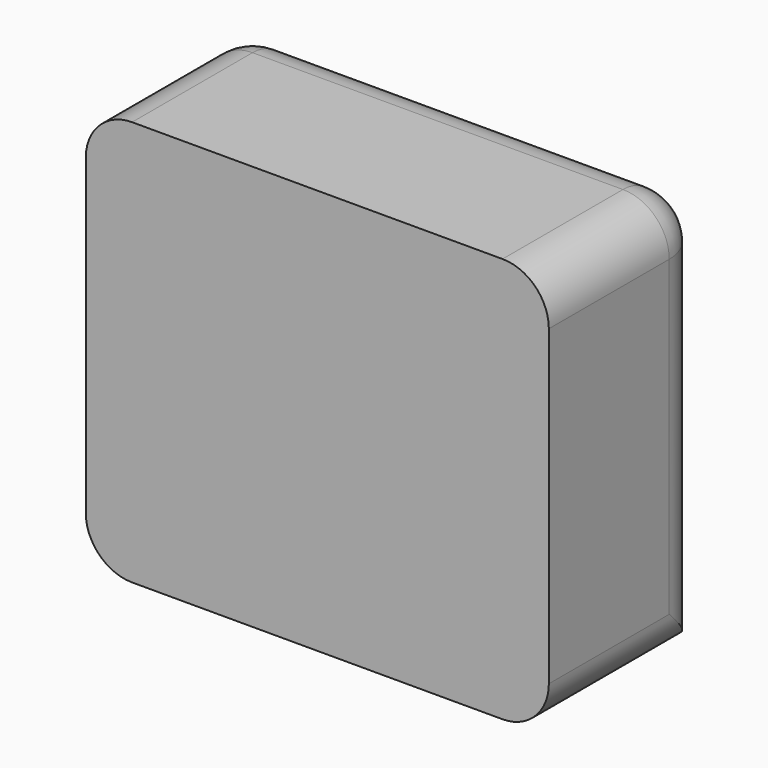
from build123d import *

# Parameters (mm, degrees)
F0_W         = 50.8
F0_H         = 44.45
F0_W_2       = 19.05
F0_H_2       = 5.08
F0_W_3       = 21.6944364339
F0_H_3       = 5.4140361476
F1_DEPTH     = 10.795
F2_W         = 50.8
F2_H         = 44.45
F3_DEPTH     = 3.81
F4_R         = 5.08
F5_SIZE      = 1.27
F6_R         = 2.54
F7_R         = 2.53999
F8_T1_DEPTH  = 52.07
F8_T3_DEPTH  = 46.99
F8_T5_DEPTH  = 40.64
F8_T8_ANGLE  = 90
F8_T10_ANGLE = 90


# Not quite as in the source:
# - a fillet or chamfer that OpenCascade refuses, or shapes differently, is made with other operations: its cross-section is extruded or revolved along the edge and cut away or added
# - a fillet or chamfer is up to 0.001 mm smaller than in the source, because OpenCascade refuses the exact size


with BuildPart() as f1:
    # F0 (on Front) → F1 (new body, symmetric)
    with BuildSketch(Plane.XZ):
        Rectangle(F0_W, F0_H)
        with Locations((-11.4416993469, -16.6936574811)):
            Rectangle(F0_W_2, F0_H_2, mode=Mode.SUBTRACT)
        with Locations((-11.4416993469, -9.0736574811)):
            Rectangle(F0_W_2, F0_H_2, mode=Mode.SUBTRACT)
        with Locations((-11.4416993469, -1.4536574811)):
            Rectangle(F0_W_2, F0_H_2, mode=Mode.SUBTRACT)
        with Locations((11.4416993469, -16.6936574811)):
            Rectangle(F0_W_2, F0_H_2, mode=Mode.SUBTRACT)
        with Locations((11.4416993469, -9.0736574811)):
            Rectangle(F0_W_2, F0_H_2, mode=Mode.SUBTRACT)
        with Locations((11.4416993469, -1.4536574811)):
            Rectangle(F0_W_2, F0_H_2, mode=Mode.SUBTRACT)
        with Locations((-11.4416993469, 6.1663425189)):
            Rectangle(F0_W_2, F0_H_2, mode=Mode.SUBTRACT)
        with Locations((-12.7639175639, 14.6224689895)):
            Rectangle(F0_W_3, F0_H_3, mode=Mode.SUBTRACT)
        with Locations((11.4416993469, 6.1663425189)):
            Rectangle(F0_W_2, F0_H_2, mode=Mode.SUBTRACT)
        with Locations((12.7639175639, 14.6224689895)):
            Rectangle(F0_W_3, F0_H_3, mode=Mode.SUBTRACT)
    extrude(amount=F1_DEPTH, both=True)

    # F2 (on face) → F3 (join)
    with BuildSketch(Plane.XZ.offset(10.795)):
        Rectangle(F2_W, F2_H)
    extrude(amount=-F3_DEPTH)

    # F4
    f4_edges = [f1.edges().sort_by_distance(p)[0] for p in [
        (25.4, 0, 22.225),
        (-25.4, 0, 22.225),
    ]]
    fillet(f4_edges, radius=F4_R)

    # F5
    f5_edges = [f1.edges().sort_by_distance(p)[0] for p in [
        (12.763918, 10.795, 11.915451),
        (-12.763918, 10.795, 11.915451),
        (-11.441699, 10.795, 3.626343),
        (11.441699, 10.795, 3.626343),
        (11.441699, 10.795, -3.993657),
        (-11.441699, 10.795, -3.993657),
        (-11.441699, 10.795, -11.613657),
        (11.441699, 10.795, -11.613657),
        (11.441699, 10.795, -19.233657),
        (-11.441699, 10.795, -19.233657),
    ]]
    chamfer(f5_edges, length=F5_SIZE)

    # F6
    f6_edges = [f1.edges().sort_by_distance(p)[0] for p in [
        (11.441699, -6.985, 3.626343),
        (-11.441699, -6.985, 3.626343),
        (-12.763918, -6.985, 11.915451),
        (12.763918, -6.985, 11.915451),
        (11.441699, -6.985, -3.993657),
        (-11.441699, -6.985, -3.993657),
        (11.441699, -6.985, -11.613657),
        (-11.441699, -6.985, -11.613657),
        (11.441699, -6.985, -19.233657),
        (-11.441699, -6.985, -19.233657),
    ]]
    fillet(f6_edges, radius=F6_R)

    # F7 (radius 2.54 in the source; OpenCascade refuses exactly that, so slightly less here)
    f7_edges = [f1.edges().sort_by_distance(p)[0] for p in [
        (11.441699, -6.985, 1.086343),
        (11.441699, -6.985, 8.706343),
        (-11.441699, -6.985, 8.706343),
        (-11.441699, -6.985, 1.086343),
        (-11.441699, -6.985, -6.533657),
        (11.441699, -6.985, -6.533657),
        (-12.763918, -6.985, 17.329487),
        (12.763918, -6.985, 17.329487),
        (11.441699, -6.985, -14.153657),
        (-11.441699, -6.985, -14.153657),
    ]]
    fillet(f7_edges, radius=F7_R)

    # F8: fillet of radius 5.08 on 4 edges, made by hand

    # F8_s2 → F8_t1 (cut)
    with BuildSketch(Plane.XY.offset(-34.925)):
        with BuildLine():
            ThreePointArc((20.32, 10.795), (23.9121024484, 9.3071024484), (25.4, 5.715))
            Line((25.4, 5.715), (25.4, 10.795))
            Line((25.4, 10.795), (20.32, 10.795))
        make_face()
        with BuildLine():
            ThreePointArc((-20.32, 10.795), (-23.9121024484, 9.3071024484), (-25.4, 5.715))
            Line((-25.4, 5.715), (-25.4, 10.795))
            Line((-25.4, 10.795), (-20.32, 10.795))
        make_face()
    extrude(amount=F8_T1_DEPTH, mode=Mode.SUBTRACT)

    # F8_s4 → F8_t3 (cut)
    with BuildSketch(Plane.XZ.offset(-23.495)):
        with BuildLine():
            ThreePointArc((-25.4, -17.145), (-23.9121024484, -20.7371024484), (-20.32, -22.225))
            Line((-20.32, -22.225), (-25.4, -22.225))
            Line((-25.4, -22.225), (-25.4, -17.145))
        make_face()
        with BuildLine():
            ThreePointArc((20.32, -22.225), (23.9121024484, -20.7371024484), (25.4, -17.145))
            Line((25.4, -17.145), (25.4, -22.225))
            Line((25.4, -22.225), (20.32, -22.225))
        make_face()
    extrude(amount=F8_T3_DEPTH, mode=Mode.SUBTRACT)

    # F8_s6 → F8_t5 (cut)
    with BuildSketch(Plane.YZ.offset(-20.32)):
        with BuildLine():
            ThreePointArc((10.795, 17.145), (9.3071024484, 20.7371024484), (5.715, 22.225))
            Line((5.715, 22.225), (10.795, 22.225))
            Line((10.795, 22.225), (10.795, 17.145))
        make_face()
    extrude(amount=F8_T5_DEPTH, mode=Mode.SUBTRACT)

    # F8_s7 → F8_t8 (revolve, cut)
    with BuildSketch(Plane.XY.offset(17.145)):
        with BuildLine():
            ThreePointArc((-20.32, 10.795), (-23.9121024484, 9.3071024484), (-25.4, 5.715))
            Line((-25.4, 5.715), (-25.4, 10.795))
            Line((-25.4, 10.795), (-20.32, 10.795))
        make_face()
    revolve(axis=Axis((-20.32, 10.795, 17.145), (0, 1, 0)), revolution_arc=F8_T8_ANGLE, mode=Mode.SUBTRACT)

    # F8_s9 → F8_t10 (revolve, cut)
    with BuildSketch(Plane.YZ.offset(20.32)):
        with BuildLine():
            ThreePointArc((10.795, 17.145), (9.3071024484, 20.7371024484), (5.715, 22.225))
            Line((5.715, 22.225), (10.795, 22.225))
            Line((10.795, 22.225), (10.795, 17.145))
        make_face()
    revolve(axis=Axis((20.32, 10.795, 17.145), (0, 1, 0)), revolution_arc=F8_T10_ANGLE, mode=Mode.SUBTRACT)


solid = f1.part
